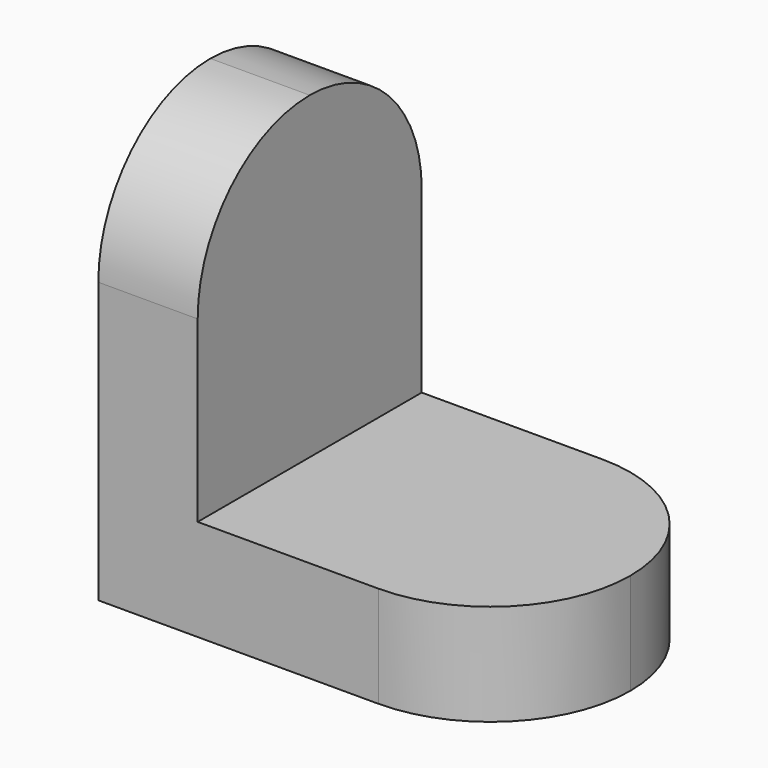
from build123d import *

# Parameters (mm, degrees)
F1_DEPTH = 38
F2_R     = 18.99999


# Not quite as in the source:
# - a fillet or chamfer is up to 0.001 mm smaller than in the source, because OpenCascade refuses the exact size


with BuildPart() as f1:
    # F0 (on Front) → F1 (new body)
    with BuildSketch(Plane.XZ):
        Polygon((-19.9589891719, 57), (-33.4447937101, 57), (-33.4447937101, 13.7555195992), (-33.4447937101, 0), (-19.9589891719, 0), (23.5552062899, 0), (23.5552062899, 13.7555195992), (-19.9589891719, 13.7555195992), align=None)
    extrude(amount=F1_DEPTH)

    # F2 (radius 19 in the source; OpenCascade refuses exactly that, so slightly less here)
    f2_edges = [f1.edges().sort_by_distance(p)[0] for p in [
        (-26.701891, -38, 57),
        (-26.701891, 0, 57),
        (23.555206, 0, 6.87776),
        (23.555206, -38, 6.87776),
    ]]
    fillet(f2_edges, radius=F2_R)


solid = f1.part
